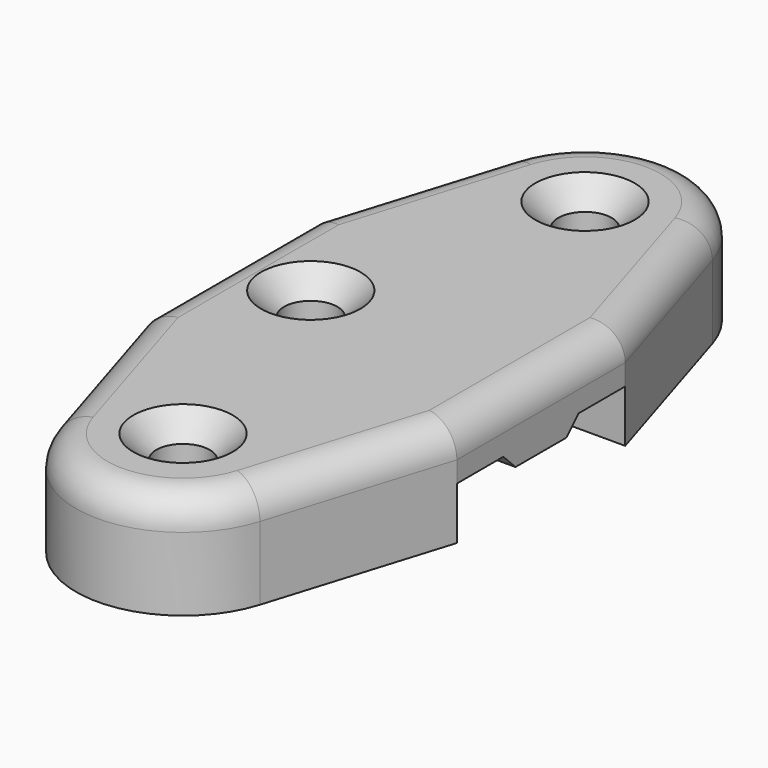
from build123d import *

# Parameters (mm, degrees)
F0_R     = 2.55
F1_DEPTH = 10
F2_W     = 20.1
F2_H     = 5
F3_DEPTH = 30.001
F5_DEPTH = 30
F6_DEPTH = 10
F7_R     = 3
F8_SIZE  = 2.2


# Not quite as in the source:
# - a feature names something its author has since deleted; it is built from what else it names


with BuildPart() as f1:
    # F0 (on Top) → F1 (new body)
    with BuildSketch(Plane.XY):
        with BuildLine():
            Line((-9.7593021288, 27.0148037464), (-15, 10.05))
            Line((-15, 10.05), (-15, -10.05))
            Line((-15, -10.05), (-9.7593021288, -27.0148037464))
            ThreePointArc((-9.7593021288, -27.0148037464), (0, -34.21435361), (9.7593021288, -27.0148037464))
            Line((9.7593021288, -27.0148037464), (15, -10.05))
            Line((15, -10.05), (15, 10.05))
            Line((15, 10.05), (9.7593021288, 27.0148037464))
            ThreePointArc((9.7593021288, 27.0148037464), (0, 34.21435361), (-9.7593021288, 27.0148037464))
        make_face()
        with Locations((-7, 0)):
            Circle(F0_R, mode=Mode.SUBTRACT)
        with Locations((0, 24)):
            Circle(F0_R, mode=Mode.SUBTRACT)
        with Locations((0, -24)):
            Circle(F0_R, mode=Mode.SUBTRACT)
    extrude(amount=F1_DEPTH)

    # F2 (on face) → F3 (cut, through all)
    with BuildSketch(Plane.YZ.offset(15)):
        with Locations((0, 2.5)):
            Rectangle(F2_W, F2_H)
    extrude(amount=-F3_DEPTH, mode=Mode.SUBTRACT)

    # F4 (on face) → F5 (join, through all)
    with BuildSketch(Plane.YZ.offset(15)):
        Polygon((3.05, 3.545), (4.5, 5), (-4.5, 5), (-3.05, 3.545), align=None)
    extrude(amount=-F5_DEPTH)

    # F0 (on Top) → F6 (cut, through all)
    with BuildSketch(Plane.XY):
        with Locations((-7, 0)):
            Circle(F0_R)
    extrude(amount=F6_DEPTH, mode=Mode.SUBTRACT)

    # F7
    f7_edges = [f1.edges().sort_by_distance(p)[0] for p in [
        (-12.379651, 18.532402, 10),
        (12.379651, 18.532402, 10),
        (12.379651, -18.532402, 10),
        (-12.379651, -18.532402, 10),
        (15, 0, 10),
        (-15, 0, 10),
    ]]
    fillet(f7_edges, radius=F7_R)

    # F8
    f8_edges = [f1.edges().sort_by_distance(p)[0] for p in [
        (-2.55, -24, 10),
        (-9.55, 0, 10),
        (-2.55, 24, 10),
    ]]
    chamfer(f8_edges, length=F8_SIZE)


solid = f1.part
